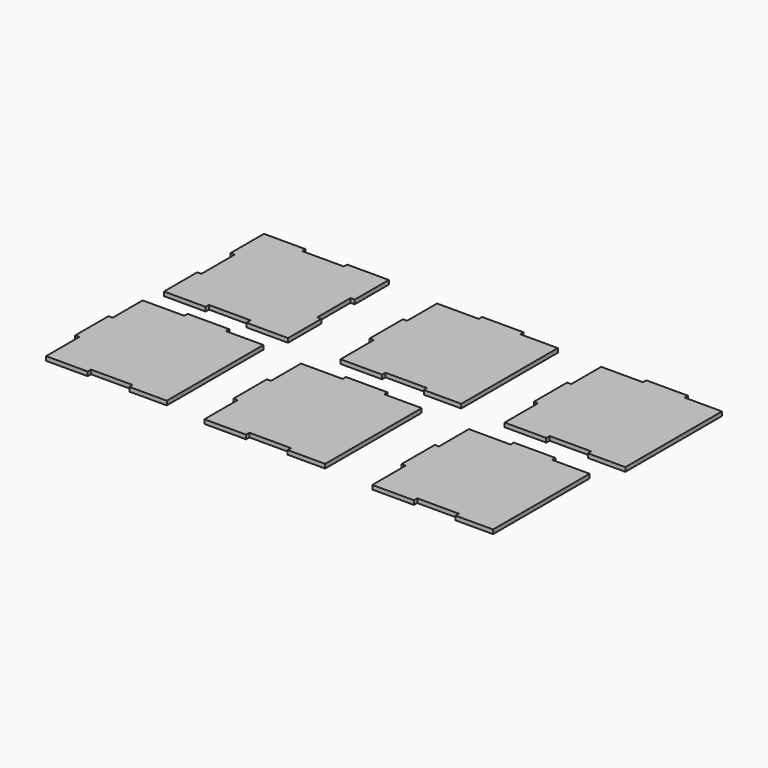
from build123d import *

# Parameters (mm, degrees)
F1_DEPTH = 5.08


# Not quite as in the source:
# - a feature names something its author has since deleted; it is built from what else it names


with BuildPart() as f1:
    # F0 (on Top) → F1 (new body)
    with BuildSketch(Plane.XY):
        Polygon((0, 152.4), (0, 101.6), (5.08, 101.6), (5.08, 50.8), (0, 50.8), (0, 0), (50.8, 0), (50.8, 5.08), (101.6, 5.08), (101.6, -1.27), (152.4, -1.27), (152.4, 49.53), (147.32, 49.53), (147.32, 100.33), (152.4, 100.33), (152.4, 152.4), (101.6, 152.4), (101.6, 147.32), (50.8, 147.32), (50.8, 152.4), align=None)
    extrude(amount=F1_DEPTH)


with BuildPart() as f1b:
    # F0 (on Top) → F1, piece 2 (new body)
    with BuildSketch(Plane.XY):
        Polygon((46.398417536, -27.047626133), (-4.401582464, -27.047626133), (-4.401582464, -72.767626133), (-9.481582464, -72.767626133), (-9.481582464, -123.567626133), (-4.401582464, -123.567626133), (-4.401582464, -174.367626133), (46.398417536, -174.367626133), (46.398417536, -169.287626133), (97.198417536, -169.287626133), (97.198417536, -174.367626133), (142.918417536, -174.367626133), (142.918417536, -27.047626133), (97.198417536, -27.047626133), (97.198417536, -21.967626133), (46.398417536, -21.967626133), align=None)
    extrude(amount=F1_DEPTH)


with BuildPart() as f1c:
    # F0 (on Top) → F1, piece 3 (new body)
    with BuildSketch(Plane.XY):
        Polygon((269.4640602303, 143.2038998055), (218.6640602303, 143.2038998055), (218.6640602303, 97.4838998055), (213.5840602303, 97.4838998055), (213.5840602303, 46.6838998055), (218.6640602303, 46.6838998055), (218.6640602303, -4.1161001945), (269.4640602303, -4.1161001945), (269.4640602303, 0.9638998055), (320.2640602303, 0.9638998055), (320.2640602303, -4.1161001945), (365.9840602303, -4.1161001945), (365.9840602303, 143.2038998055), (320.2640602303, 143.2038998055), (320.2640602303, 148.2838998055), (269.4640602303, 148.2838998055), align=None)
    extrude(amount=F1_DEPTH)


with BuildPart() as f1d:
    # F0 (on Top) → F1, piece 4 (new body)
    with BuildSketch(Plane.XY):
        Polygon((473.199620409, 138.8687571335), (422.399620409, 138.8687571335), (422.399620409, 93.1487571335), (417.319620409, 93.1487571335), (417.319620409, 42.3487571335), (422.399620409, 42.3487571335), (422.399620409, -8.4512428665), (473.199620409, -8.4512428665), (473.199620409, -3.3712428665), (523.999620409, -3.3712428665), (523.999620409, -8.4512428665), (569.719620409, -8.4512428665), (569.719620409, 138.8687571335), (523.999620409, 138.8687571335), (523.999620409, 143.9487571335), (473.199620409, 143.9487571335), align=None)
    extrude(amount=F1_DEPTH)


with BuildPart() as f1e:
    # F0 (on Top) → F1, piece 5 (new body)
    with BuildSketch(Plane.XY):
        Polygon((455.1379527283, -40.3170431209), (404.3379527283, -40.3170431209), (404.3379527283, -86.0370431209), (399.2579527283, -86.0370431209), (399.2579527283, -136.8370431209), (404.3379527283, -136.8370431209), (404.3379527283, -187.6370431209), (455.1379527283, -187.6370431209), (455.1379527283, -182.5570431209), (505.9379527283, -182.5570431209), (505.9379527283, -187.6370431209), (551.6579527283, -187.6370431209), (551.6579527283, -40.3170431209), (505.9379527283, -40.3170431209), (505.9379527283, -35.2370431209), (455.1379527283, -35.2370431209), align=None)
    extrude(amount=F1_DEPTH)


with BuildPart() as f1f:
    # F0 (on Top) → F1, piece 6 (new body)
    with BuildSketch(Plane.XY):
        Polygon((245.6226493549, -34.536860342), (194.8226493549, -34.536860342), (194.8226493549, -80.256860342), (189.7426493549, -80.256860342), (189.7426493549, -131.056860342), (194.8226493549, -131.056860342), (194.8226493549, -181.856860342), (245.6226493549, -181.856860342), (245.6226493549, -176.776860342), (296.4226493549, -176.776860342), (296.4226493549, -181.856860342), (342.1426493549, -181.856860342), (342.1426493549, -34.536860342), (296.4226493549, -34.536860342), (296.4226493549, -29.456860342), (245.6226493549, -29.456860342), align=None)
    extrude(amount=F1_DEPTH)


solid = Compound([f1.part, f1b.part, f1c.part, f1d.part, f1e.part, f1f.part])
